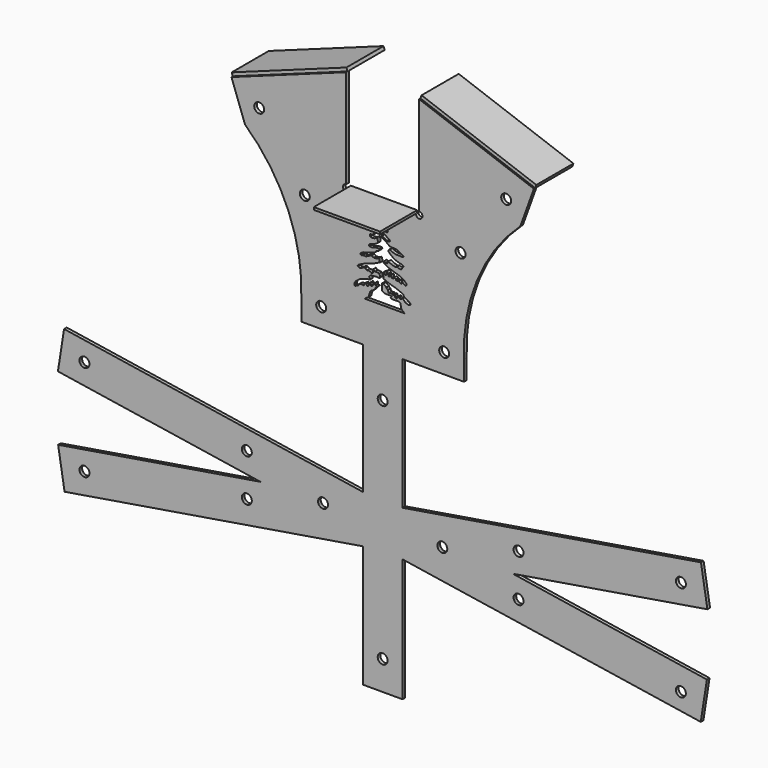
from build123d import *

# Parameters (mm, degrees)
F0_R     = 9.525
F0_R_2   = 3.175
F1_DEPTH = 3.175
F2_DEPTH = 88.9
F0_W     = 127
F0_H     = 4.7752
F3_DEPTH = 88.9


# Not quite as in the source:
# - a feature names something its author has since deleted; it is built from what else it names


with BuildPart() as f1:
    # F0 (on Front) → F1 (new body, symmetric)
    with BuildSketch(Plane.XZ):
        Polygon((-69.85, 303.926875), (-203.2, 255.5875), (-69.85, 255.5875), align=None)
        with BuildLine():
            Line((-167.3808159173, -1.6199540129), (-203.2, 255.5875))
            Line((-203.2, 255.5875), (-203.2, 78.7780769081))
            ThreePointArc((-203.2, 78.7780769081), (-182.9956492828, 39.6036195315), (-168.1761064252, -1.908246822))
            Line((-168.1761064252, -1.908246822), (-167.3808159173, -1.6199540129))
        make_face()
        with BuildLine():
            Line((-69.85, 255.5875), (-203.2, 255.5875))
            Line((-203.2, 255.5875), (-167.3808159173, -1.6199540129))
            Line((-167.3808159173, -1.6199540129), (-168.1761064252, -1.908246822))
            ThreePointArc((-168.1761064252, -1.908246822), (-157.8501469155, -53.8850159886), (-155.95205801, -106.8435585601))
            Line((-155.95205801, -106.8435585601), (-155.95205801, -144.9435585601))
            Line((-155.95205801, -144.9435585601), (-38.1, -144.9435585601))
            Line((-38.1, -144.9435585601), (0, -144.9435585601))
            Line((0, -144.9435585601), (38.1, -144.9435585601))
            Line((38.1, -144.9435585601), (155.95205801, -144.9435585601))
            Line((155.95205801, -144.9435585601), (155.95205801, -106.8435585601))
            ThreePointArc((155.95205801, -106.8435585601), (157.8501469155, -53.8850159886), (168.1761064252, -1.908246822))
            Line((168.1761064252, -1.908246822), (167.3808159173, -1.6199540129))
            Line((167.3808159173, -1.6199540129), (203.2, 255.5875))
            Line((203.2, 255.5875), (69.85, 255.5875))
            Line((69.85, 255.5875), (69.85, 114.9223))
            ThreePointArc((69.85, 114.9223), (74.3401280605, 113.0624280605), (76.2, 108.5723))
            ThreePointArc((76.2, 108.5723), (69.85, 102.2223), (63.5, 108.5723))
            Line((63.5, 108.5723), (-63.5, 108.5723))
            ThreePointArc((-63.5, 108.5723), (-74.3401280605, 104.0821719395), (-69.85, 114.9223))
            Line((-69.85, 114.9223), (-69.85, 255.5875))
        make_face()
        with Locations((-117.856, -107.2179209328)):
            Circle(F0_R, mode=Mode.SUBTRACT)
        with Locations((0, -106.8435585601)):
            Circle(F0_R_2, mode=Mode.SUBTRACT)
        with Locations((-100.6744361574, -17.9435585601)):
            Circle(F0_R_2, mode=Mode.SUBTRACT)
        Polygon((-34.7350827502, -66.5424876551), (-31.054901992, -63.8737194877), (-27.094953795, -61.4368282895), (-23.7442283975, -50.6168401842), (-21.6119485991, -48.7891680603), (-17.0427757399, -46.3522805874), (-14.9104959415, -43.9153893892), (-13.0828275429, -40.5646621291), (-10.1018175111, -38.4779572487), (-11.5208746865, -38.4779572487), (-13.9577658847, -37.564124912), (-14.2623763531, -33.2995653152), (-15.785433352, -34.8226204515), (-17.0038808137, -36.6502888501), (-18.2223245502, -38.1733439863), (-19.4407720119, -40.3056256473), (-22.7914974093, -40.9148484468), (-23.0961069465, -38.7825705111), (-23.0961069465, -35.9453856945), (-24.5961938053, -36.2300090492), (-24.619165808, -36.3456755877), (-25.837611407, -38.4779572487), (-27.0560570061, -42.7425168455), (-29.4929482043, -43.6563529074), (-31.62522614, -41.5240712464), (-32.2344489396, -39.6964028478), (-34.671343863, -40.9148484468), (-36.1943989992, -44.5701815188), (-40.1543490589, -44.2655719817), (-44.1142953932, -44.5701815188), (-46.8557998538, -48.2255220413), (-53.2526373863, -51.271636039), (-54.1664734483, -48.5301353037), (-53.5572506487, -45.4840175807), (-51.4249689877, -42.437903583), (-44.4189086556, -36.9548983872), (-32.539062202, -32.6903387904), (-23.4007202089, -30.5580608547), (-24.619165808, -29.0350038558), (-26.1422228068, -26.2935012579), (-23.7053316087, -24.1612195969), (-18.5269378126, -22.9427739978), (-13.3485421538, -22.3335511982), (-6.9517027587, -22.638162598), (-5.1240348257, -21.7243302613), (-5.1240348257, -18.3736030012), (-6.3424808905, -15.0228776038), (-10.3024281561, -14.4136548042), (-14.871600084, -14.4136548042), (-17.9891549051, -11.3546038046), (-19.4676760584, -13.0302608013), (-19.4407720119, -13.1952101365), (-18.2223245502, -18.0689916015), (-20.6592157483, -19.5920486003), (-23.4007202089, -17.7643802017), (-25.837611407, -16.8505460024), (-30.1021710038, -17.1551574022), (-33.4528945386, -14.4136548042), (-36.4990122616, -14.7182652727), (-43.2004630566, -18.0689916015), (-46.8557998538, -16.5459346026), (-48.0742454529, -15.0228776038), (-45.0281314552, -12.2813750058), (-35.8897894621, -8.0168154091), (-20.6592157483, -2.8384211473), (-9.3885958195, 1.7307501985), (-8.4747597575, 2.949195914), (-5.4286457598, 3.5584187135), (-5.7332566939, 6.6045327112), (-6.9517027587, 10.5644809082), (-8.4747597575, 9.9552581087), (-12.1300965548, 8.4322011098), (-17.0038808137, 8.1275897101), (-21.2684404105, 10.2598704398), (-25.5330000073, 8.7368125096), (-32.2344489396, 5.3860871121), (-37.7174578607, 5.6906985119), (-40.1543490589, 4.4722529128), (-42.8958497941, 5.3860871121), (-42.591240257, 7.8229783103), (-36.1943989992, 11.1737037078), (-27.6652798057, 13.6105958372), (-16.0900466144, 16.9613212347), (-12.1300965548, 20.9212694317), (-8.1701492891, 22.4443264306), (-5.7332566939, 24.8812176287), (-6.3424808905, 26.7088860273), (-10.3024281561, 27.0134974271), (-13.0439316854, 26.4042746276), (-19.745381549, 24.2719948292), (-25.2283886075, 24.5766080916), (-26.7514456064, 27.0134974271), (-24.619165808, 28.8411676884), (-19.745381549, 30.0596132874), (-13.6531544849, 32.8011140227), (-8.7793711573, 36.1518375576), (-10.3024281561, 44.3763509393), (-15.723541379, 41.2169061601), (-20.3084610403, 40.5801124871), (-23.8745100796, 41.598983109), (-24.0018684417, 45.5471090972), (-19.4169487804, 46.8206964433), (-14.9655133062, 49.0394322011), (-23.0358543025, 57.109766468), (-21.5489892105, 58.5966315599), (-15.152150281, 59.2058506342), (-11.8014251164, 62.2519646319), (-14.8475370186, 64.9934690924), (-18.1982647444, 67.1257507535), (-18.5028761441, 69.2580324145), (-14.8475370186, 70.1718684765), (-10.8875896365, 71.0856970878), (-9.6691433389, 73.2179750236), (-13.6290932822, 72.6087559493), (-16.0659830833, 73.8272015484), (-13.9337042163, 76.5687022837), (-10.5829787024, 79.9194295438), (-6.623028992, 83.8793758782), (-6.3184180579, 88.7531582745), (-4.186138958, 90.5808303984), (-2.0538600909, 90.5808303984), (-0.8354065756, 87.534720126), (-2.6630749742, 79.3102104696), (-3.881521039, 74.1318185361), (-3.2722996364, 68.0395868154), (1.6014827599, 65.9073088797), (7.6937116866, 63.7750309439), (10.1306047474, 60.7289169462), (9.2167686855, 58.9012448223), (5.2568195572, 59.2058543595), (-1.4446312378, 59.5104676219), (-1.4446312378, 57.0735764237), (3.4291539525, 54.3320756884), (10.7398256843, 49.7629065545), (14.699775744, 46.4121792944), (13.1767187451, 44.8891204329), (8.3029344862, 44.8891204329), (4.0383758207, 47.021402094), (-1.1400179754, 50.3721256288), (-3.2722996364, 50.0675160917), (-3.2722996364, 48.239847693), (3.1245406901, 44.5845108958), (7.9983249491, 41.5383968981), (13.1767187451, 37.2738354387), (20.4873923396, 36.6646145018), (26.27500521, 36.360003102), (40.4856278915, 29.2077419829), (39.2671860178, 27.0754621846), (33.4795694221, 27.380075447), (25.2550616283, 27.380075447), (17.335161509, 29.5123533827), (13.9844389055, 31.9492445809), (11.8521572445, 31.0354103816), (10.9383216482, 28.2939077836), (15.202882642, 23.7247367871), (22.8181685675, 18.2417315912), (32.8703410347, 14.8910061938), (37.7441271563, 13.9771719945), (40.1810183544, 11.540279865), (35.0846797228, 5.0814799033), (30.5155068636, 5.9953141026), (27.4693928659, 6.9091478363), (23.8140560687, 5.9953141026), (20.4633288085, 6.9091478363), (16.5033787489, 8.1275943667), (10.7157630846, 10.8690969646), (9.801927954, 9.0414276347), (9.4973193482, 6.9091478363), (5.5373697542, 6.9091478363), (3.100479953, 9.0414276347), (1.2728092261, 7.2137597017), (3.100479953, 4.4722571038), (10.1065412164, 0.8169198991), (21.9863858074, -3.1430283561), (33.2570075989, -6.798365619), (40.8722944558, -11.0629247501), (45.1368540525, -15.0228738785), (45.7460805774, -18.3735992759), (43.9184084535, -19.592044875), (39.9584583938, -17.1551536769), (36.6305209872, -14.4322942851), (37.102624774, -17.7370272577), (35.3892855346, -18.9828220755), (32.6477847993, -17.7643764764), (30.8201164007, -15.9367080778), (25.3371130675, -16.2413194776), (25.3371130675, -14.4136510789), (21.9863858074, -12.5859826803), (21.6817781329, -14.1090396792), (20.4633288085, -15.0228738785), (17.4172148108, -14.7182624787), (15.894157812, -10.7583133504), (14.3710998818, -11.0629247501), (14.066491276, -13.8044282794), (11.934212409, -14.1090396792), (10.7157630846, -12.8905931488), (11.0203772783, -9.5398677513), (7.9742623493, -6.798365619), (5.8419806883, -7.7121998183), (7.9742623493, -10.7583133504), (6.7558162846, -13.4998159483), (4.0143127553, -13.4998159483), (1.8820336554, -9.8444800824), (1.5774228377, -11.672148481), (0.9681983502, -14.7182624787), (1.8820336554, -21.4197132736), (4.0143127553, -22.333547473), (11.6295991465, -25.3796614707), (25.946335867, -29.6442210674), (40.5676811934, -35.7364490628), (39.9584583938, -37.8687307239), (42.9591350257, -39.7909916937), (50.2884611487, -44.0955162048), (50.315245986, -44.2655682564), (53.6659732461, -46.7024594545), (52.7521446347, -49.4439639151), (49.4014173746, -50.0531904399), (43.613795191, -47.9209087789), (39.3492355943, -43.6563491821), (37.8261804581, -43.0471226573), (34.7800664604, -44.8747947812), (33.2570075989, -44.8747947812), (31.1247296631, -43.9609587193), (29.6016726643, -42.1332903206), (28.6878366023, -43.3517359197), (28.128749868, -44.6562678347), (45.9769143052, -54.0322429171), (38.0124577389, -63.3241170279), (41.8898276985, -66.5983408689), (33.8273354722, -66.5424876551), align=None, mode=Mode.SUBTRACT)
        with Locations((-149.225, 70.5820790672)):
            Circle(F0_R, mode=Mode.SUBTRACT)
        with Locations((117.856, -107.2179209328)):
            Circle(F0_R, mode=Mode.SUBTRACT)
        with Locations((100.6744361574, -17.9435585601)):
            Circle(F0_R_2, mode=Mode.SUBTRACT)
        with Locations((149.225, 70.5820790672)):
            Circle(F0_R, mode=Mode.SUBTRACT)
        with BuildLine():
            Line((-203.2, 78.7780769081), (-203.2, 255.5875))
            Line((-203.2, 255.5875), (-289.7688754486, 224.2062826499))
            Line((-289.7688754486, 224.2062826499), (-263.7999669887, 152.5679144845))
            ThreePointArc((-263.7999669887, 152.5679144845), (-230.8249337186, 117.8698826041), (-203.2, 78.7780769081))
        make_face()
        with Locations((-236.6264, 189.4540790672)):
            Circle(F0_R, mode=Mode.SUBTRACT)
        Polygon((69.85, 303.926875), (69.85, 255.5875), (203.2, 255.5875), align=None)
        with BuildLine():
            Line((289.7688754486, 224.2062826499), (203.2, 255.5875))
            Line((203.2, 255.5875), (203.2, 78.7780769081))
            ThreePointArc((203.2, 78.7780769081), (230.8249337186, 117.8698826041), (263.7999669887, 152.5679144845))
            Line((263.7999669887, 152.5679144845), (289.7688754486, 224.2062826499))
        make_face()
        with Locations((236.6264, 189.4540790672)):
            Circle(F0_R, mode=Mode.SUBTRACT)
        with BuildLine():
            Line((203.2, 78.7780769081), (203.2, 255.5875))
            Line((203.2, 255.5875), (167.3808159173, -1.6199540129))
            Line((167.3808159173, -1.6199540129), (168.1761064252, -1.908246822))
            ThreePointArc((168.1761064252, -1.908246822), (182.9956492828, 39.6036195315), (203.2, 78.7780769081))
        make_face()
        with BuildLine():
            Line((0, -144.9435585601), (-38.1, -144.9435585601))
            Line((-38.1, -144.9435585601), (-38.1, -302.1797800928))
            Line((-38.1, -302.1797800928), (0, -308.0801984275))
            Line((0, -308.0801984275), (0, -236.4149232149))
            ThreePointArc((0, -236.4149232149), (-9.525, -226.8899232149), (0, -217.3649232149))
            Line((0, -217.3649232149), (0, -144.9435585601))
        make_face()
        with BuildLine():
            Line((38.1, -144.9435585601), (0, -144.9435585601))
            Line((0, -144.9435585601), (0, -217.3649232149))
            ThreePointArc((0, -217.3649232149), (6.7351920908, -220.1547311241), (9.525, -226.8899232149))
            ThreePointArc((9.525, -226.8899232149), (6.7351920908, -233.6251153057), (0, -236.4149232149))
            Line((0, -236.4149232149), (0, -308.0801984275))
            Line((0, -308.0801984275), (13.9258963624, -310.2368549689))
            Line((13.9258963624, -310.2368549689), (38.1, -306.2673607271))
            Line((38.1, -306.2673607271), (38.1, -144.9435585601))
        make_face()
        Polygon((0, -308.0801984275), (-38.1, -302.1797800928), (-38.1, -318.7797361912), (0, -312.5235484592), align=None)
        Polygon((13.9258963624, -310.2368549689), (0, -308.0801984275), (0, -312.5235484592), align=None)
        Polygon((0, -312.5235484592), (-38.1, -318.7797361912), (-38.1, -393.7680730425), (0, -399.6684913773), align=None)
        Polygon((-38.1, -393.7680730425), (-203.2, -368.199593592), (-203.2, -435.4097823141), (-38.1, -408.2996354752), align=None)
        Polygon((-203.2, -435.4097823141), (-203.2, -368.199593592), (-273.1208288678, -357.3711909507), (-514.7860304257, -397.0536809572), (-234.221854538, -440.5037074003), align=None)
        with Locations((-260.35, -396.7779209328)):
            Circle(F0_R, mode=Mode.SUBTRACT)
        Polygon((-514.7860304257, -397.0536809572), (-273.1208288678, -357.3711909507), (-586.9146884545, -308.7749956111), (-610.6381813392, -305.1010183833), (-622.3, -380.4033555683), (-596.622441127, -384.3799523968), align=None)
        with Locations((-571.5, -348.5179209328)):
            Circle(F0_R, mode=Mode.SUBTRACT)
        Polygon((38.1, -313.9806167623), (38.1, -306.2673607271), (13.9258963624, -310.2368549689), align=None)
        Polygon((38.1, -313.9806167623), (13.9258963624, -310.2368549689), (0, -312.5235484592), (0, -399.6684913773), (7.4433470199, -400.8212173938), (38.1, -395.7872600111), align=None)
        Polygon((0, -399.6684913773), (-38.1, -393.7680730425), (-38.1, -408.2996354752), (0, -402.0434477432), align=None)
        Polygon((-38.1, -408.2996354752), (-203.2, -435.4097823141), (-203.2, -445.3079572505), (-38.1, -470.8764367011), (-38.1, -437.4179209328), align=None)
        with BuildLine():
            ThreePointArc((-123.825, -437.4179209328), (-114.3, -427.8929209328), (-104.775, -437.4179209328))
            ThreePointArc((-104.775, -437.4179209328), (-114.3, -446.9429209328), (-123.825, -437.4179209328))
        make_face(mode=Mode.SUBTRACT)
        Polygon((-203.2, -445.3079572505), (-203.2, -435.4097823141), (-234.221854538, -440.5037074003), align=None)
        Polygon((7.4433470199, -400.8212173938), (0, -399.6684913773), (0, -402.0434477432), align=None)
        Polygon((0, -402.0434477432), (-38.1, -408.2996354752), (-38.1, -437.4179209328), (0, -437.4179209328), align=None)
        Polygon((-38.1, -470.8764367011), (-203.2, -445.3079572505), (-203.2, -512.630242943), (-38.1, -485.5200961042), align=None)
        Polygon((-203.2, -512.630242943), (-203.2, -445.3079572505), (-234.221854538, -440.5037074003), (-520.99789372, -487.5935955413), (-278.9813692229, -525.0738773906), align=None)
        with Locations((-260.35, -478.0579209328)):
            Circle(F0_R, mode=Mode.SUBTRACT)
        Polygon((203.2, -368.6771131723), (38.1, -395.7872600111), (38.1, -405.568909712), (203.2, -431.1373891626), align=None)
        Polygon((38.1, -405.568909712), (38.1, -395.7872600111), (7.4433470199, -400.8212173938), align=None)
        Polygon((38.1, -405.568909712), (7.4433470199, -400.8212173938), (0, -402.0434477432), (0, -437.4179209328), (38.1, -437.4179209328), align=None)
        Polygon((0, -437.4179209328), (-38.1, -437.4179209328), (-38.1, -470.8764367011), (0, -476.7768550359), align=None)
        Polygon((294.4900722501, -353.686881412), (203.2, -368.6771131723), (203.2, -431.1373891626), (249.459871517, -438.301499243), (535.1558805077, -391.3889568141), (536.5065967472, -391.1671632612), align=None)
        with Locations((260.35, -396.7779209328)):
            Circle(F0_R, mode=Mode.SUBTRACT)
        Polygon((446.7980133413, -328.6772469619), (294.4900722501, -353.686881412), (536.5065967472, -391.1671632612), (622.3, -377.0795087488), (609.9529743206, -301.8864840931), align=None)
        with Locations((571.5, -348.5179209328)):
            Circle(F0_R, mode=Mode.SUBTRACT)
        Polygon((0, -476.7768550359), (-38.1, -470.8764367011), (-38.1, -485.5200961042), (0, -479.2639083722), align=None)
        Polygon((-278.9813692229, -525.0738773906), (-520.99789372, -487.5935955413), (-621.9470256794, -504.1698874291), (-609.6, -579.3629120848), align=None)
        with Locations((-571.5, -532.6679209328)):
            Circle(F0_R, mode=Mode.SUBTRACT)
        Polygon((203.2, -431.1373891626), (38.1, -405.568909712), (38.1, -437.4179209328), (38.1, -473.0077206401), (203.2, -445.8975738013), align=None)
        with BuildLine():
            ThreePointArc((123.825, -437.4179209328), (114.3, -446.9429209328), (104.775, -437.4179209328))
            ThreePointArc((104.775, -437.4179209328), (114.3, -427.8929209328), (123.825, -437.4179209328))
        make_face(mode=Mode.SUBTRACT)
        Polygon((38.1, -437.4179209328), (0, -437.4179209328), (0, -476.7768550359), (7.7946699591, -477.9839892495), (38.1, -473.0077206401), align=None)
        Polygon((249.459871517, -438.301499243), (203.2, -431.1373891626), (203.2, -445.8975738013), align=None)
        Polygon((0, -479.2639083722), (-38.1, -485.5200961042), (-38.1, -562.3783615759), (0, -568.2787799107), align=None)
        Polygon((7.7946699591, -477.9839892495), (0, -476.7768550359), (0, -479.2639083722), align=None)
        Polygon((249.459871517, -438.301499243), (203.2, -445.8975738013), (203.2, -508.2457528212), (287.7271166274, -521.3361819218), (550.0512124119, -561.9614287568), (609.6, -571.1835483919), (621.2618186608, -495.8812112069), (562.2734502701, -486.7458818003), align=None)
        with Locations((571.5, -532.6679209328)):
            Circle(F0_R, mode=Mode.SUBTRACT)
        with Locations((260.35, -478.0579209328)):
            Circle(F0_R, mode=Mode.SUBTRACT)
        Polygon((203.2, -508.2457528212), (203.2, -445.8975738013), (38.1, -473.0077206401), (38.1, -482.6772733706), align=None)
        Polygon((0, -568.2787799107), (-38.1, -562.3783615759), (-38.1, -574.8384288984), (0, -568.5822411664), align=None)
        Polygon((7.7946699591, -477.9839892495), (0, -479.2639083722), (0, -568.2787799107), (0.9510774453, -568.4260700628), (38.1, -562.3260534343), (38.1, -482.6772733706), align=None)
        Polygon((38.1, -473.0077206401), (7.7946699591, -477.9839892495), (38.1, -482.6772733706), align=None)
        Polygon((0.9510774453, -568.4260700628), (0, -568.2787799107), (0, -568.5822411664), align=None)
        with BuildLine():
            Line((0, -568.5822411664), (-38.1, -574.8384288984))
            Line((-38.1, -574.8384288984), (-38.1, -718.9269661903))
            Line((-38.1, -718.9269661903), (0, -718.9269661903))
            Line((0, -718.9269661903), (0, -672.5687374115))
            ThreePointArc((0, -672.5687374115), (-9.525, -663.0437374115), (0, -653.5187374115))
            Line((0, -653.5187374115), (0, -568.5822411664))
        make_face()
        with BuildLine():
            Line((38.1, -574.1791982454), (0.9510774453, -568.4260700628))
            Line((0.9510774453, -568.4260700628), (0, -568.5822411664))
            Line((0, -568.5822411664), (0, -653.5187374115))
            ThreePointArc((0, -653.5187374115), (6.7351920908, -656.3085453207), (9.525, -663.0437374115))
            ThreePointArc((9.525, -663.0437374115), (6.7351920908, -669.7789295023), (0, -672.5687374115))
            Line((0, -672.5687374115), (0, -718.9269661903))
            Line((0, -718.9269661903), (38.1, -718.9269661903))
            Line((38.1, -718.9269661903), (38.1, -574.1791982454))
        make_face()
        Polygon((38.1, -562.3260534343), (0.9510774453, -568.4260700628), (38.1, -574.1791982454), align=None)
        with Locations((-100.6744361574, -17.9435585601)):
            Circle(F0_R_2)
        with Locations((0, -106.8435585601)):
            Circle(F0_R_2)
        with Locations((100.6744361574, -17.9435585601)):
            Circle(F0_R_2)
        Polygon((15.1375159118, -48.6213441242), (17.110209886, -50.3122231965), (31.6950575365, -50.3122231965), (33.8273354722, -51.5306687955), (35.86428985, -61.5101084113), (38.0124577389, -63.3241170279), (45.9769143052, -54.0322429171), (28.128749868, -44.6562678347), (27.7740005404, -45.4840138555), (26.2509435415, -46.3978499174), (23.8140560687, -45.7886271179), (23.5094428062, -43.3517359197), (22.985438002, -41.9543897751), (21.9221994703, -41.3958506595), (20.4633288085, -42.4378998578), (18.6356622726, -43.0471226573), (17.7218280733, -41.5240675211), (14.1694936901, -41.3663946092), (14.066491276, -41.5240675211), (11.934212409, -42.4378998578), (11.0203772783, -40.9148447216), (9.801927954, -37.5641174614), (6.7558162846, -34.8226167262), (6.0713343204, -36.3456718624), (6.0713343204, -40.8503381199), (11.4241298027, -45.4384445254), (16.1598724229, -45.4384445254), (17.3622787846, -47.055362076), (15.5039382083, -48.1703638141), align=None)
        Polygon((4.2800278319, -45.4384445254), (11.4241298027, -45.4384445254), (6.0713343204, -40.8503381199), (6.0713343204, -36.3456718624), (6.7558162846, -34.8226167262), (7.3218145442, -33.7259949865), (0.6246915003, -30.2078708117), (-1.5075901607, -30.2078708117), (-1.5075901607, -42.0877172653), align=None)
    extrude(amount=F1_DEPTH, both=True)

    # F0 (on Front) → F2 (join)
    with BuildSketch(Plane.XZ):
        Polygon((-289.7688754486, 224.2062826499), (-203.2, 255.5875), (-69.85, 303.926875), (-72.014075705, 309.8967390138), (-291.9329511536, 230.1761466637), align=None)
        Polygon((72.014075705, 309.8967390138), (69.85, 303.926875), (203.2, 255.5875), (289.7688754486, 224.2062826499), (291.9329511536, 230.1761466637), align=None)
    extrude(amount=-F2_DEPTH)

    # F0 (on Front) → F3 (join)
    with BuildSketch(Plane.XZ):
        with Locations((0, 110.9599)):
            Rectangle(F0_W, F0_H)
    extrude(amount=F3_DEPTH)


solid = f1.part
